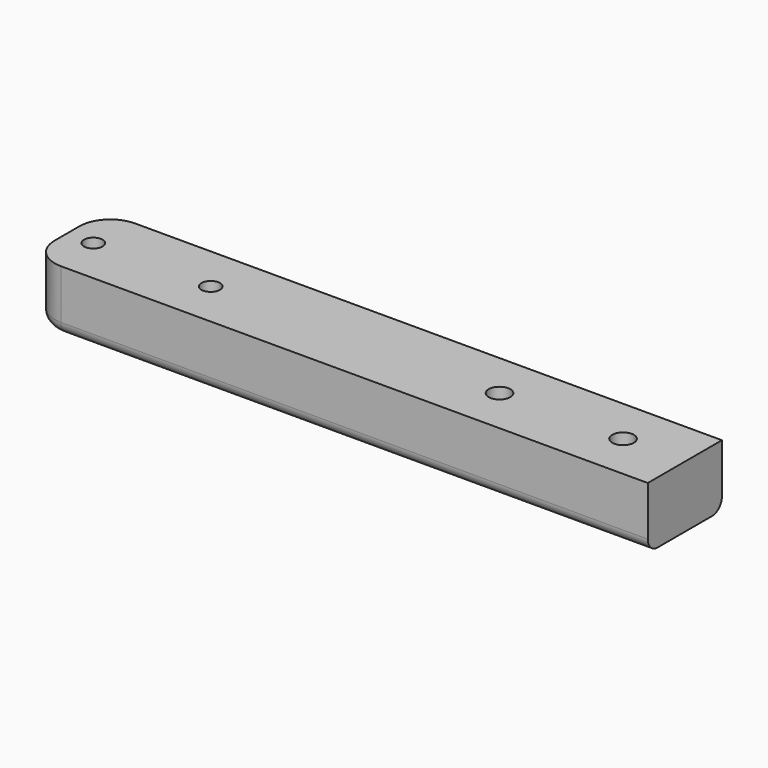
from build123d import *

# Parameters (mm, degrees)
F0_W        = 60
F0_H        = 15
F0_R        = 1.5
F0_W_2      = 40
F0_R_2      = 1.75
F1_DEPTH    = 5
F2_T        = -2
F3_R        = 5
F4_R        = 5
F5_T1_DEPTH = 100
F5_T3_DEPTH = 5
F5_T6_ANGLE = 90
F5_T8_ANGLE = 90


# Not quite as in the source:
# - a fillet or chamfer that OpenCascade refuses, or shapes differently, is made with other operations: its cross-section is extruded or revolved along the edge and cut away or added


with BuildPart() as f1:
    # F0 (on Top) → F1 (new body, symmetric)
    with BuildSketch(Plane.XY):
        with Locations((-20, 0)):
            Rectangle(F0_W, F0_H)
        with Locations((-45.75, 0)):
            Circle(F0_R, mode=Mode.SUBTRACT)
        with Locations((-26.75, 0)):
            Circle(F0_R, mode=Mode.SUBTRACT)
        with Locations((30, 0)):
            Rectangle(F0_W_2, F0_H)
        with Locations((20, 0)):
            Circle(F0_R_2, mode=Mode.SUBTRACT)
        with Locations((40, 0)):
            Circle(F0_R_2, mode=Mode.SUBTRACT)
    extrude(amount=F1_DEPTH, both=True)

    # F2
    f2_openings = [f1.faces().sort_by_distance(p)[0] for p in [
        (-0.04418, 0, -5),
    ]]
    offset(amount=F2_T, openings=f2_openings, kind=Kind.INTERSECTION)

    # F3
    f3_edges = [f1.edges().sort_by_distance(p)[0] for p in [
        (-50, -7.5, 0),
    ]]
    fillet(f3_edges, radius=F3_R)

    # F4
    f4_edges = [f1.edges().sort_by_distance(p)[0] for p in [
        (-50, 7.5, 0),
    ]]
    fillet(f4_edges, radius=F4_R)

    # F5: fillet of radius 2 on 1 edges, made by hand

    # F5_s2 → F5_t1 (cut)
    with BuildSketch(Plane.YZ.offset(-45)):
        with BuildLine():
            ThreePointArc((-5.5, -5), (-6.9142135624, -4.4142135624), (-7.5, -3))
            Line((-7.5, -3), (-7.5, -5))
            Line((-7.5, -5), (-5.5, -5))
        make_face()
        with BuildLine():
            ThreePointArc((5.5, -5), (6.9142135624, -4.4142135624), (7.5, -3))
            Line((7.5, -3), (7.5, -5))
            Line((7.5, -5), (5.5, -5))
        make_face()
    extrude(amount=F5_T1_DEPTH, mode=Mode.SUBTRACT)

    # F5_s4 → F5_t3 (cut)
    with BuildSketch(Plane.XZ.offset(-2.5)):
        with BuildLine():
            ThreePointArc((-50, -3), (-49.4142135624, -4.4142135624), (-48, -5))
            Line((-48, -5), (-50, -5))
            Line((-50, -5), (-50, -3))
        make_face()
    extrude(amount=F5_T3_DEPTH, mode=Mode.SUBTRACT)

    # F5_s5 → F5_t6 (revolve, cut)
    with BuildSketch(Plane.XZ.offset(2.5)):
        with BuildLine():
            ThreePointArc((-48, -5), (-49.4142135624, -4.4142135624), (-50, -3))
            Line((-50, -3), (-50, -5))
            Line((-50, -5), (-48, -5))
        make_face()
    revolve(axis=Axis((-45, -2.5, -5), (0, 0, 1)), revolution_arc=F5_T6_ANGLE, mode=Mode.SUBTRACT)

    # F5_s7 → F5_t8 (revolve, cut)
    with BuildSketch(Plane.XZ.offset(-2.5)):
        with BuildLine():
            ThreePointArc((-48, -5), (-49.4142135624, -4.4142135624), (-50, -3))
            Line((-50, -3), (-50, -5))
            Line((-50, -5), (-48, -5))
        make_face()
    revolve(axis=Axis((-45, 2.5, -5), (0, 0, -1)), revolution_arc=F5_T8_ANGLE, mode=Mode.SUBTRACT)


with BuildPart() as f6_1:
    # F6: copy of F1
    add(f1.part)


solid = f6_1.part
